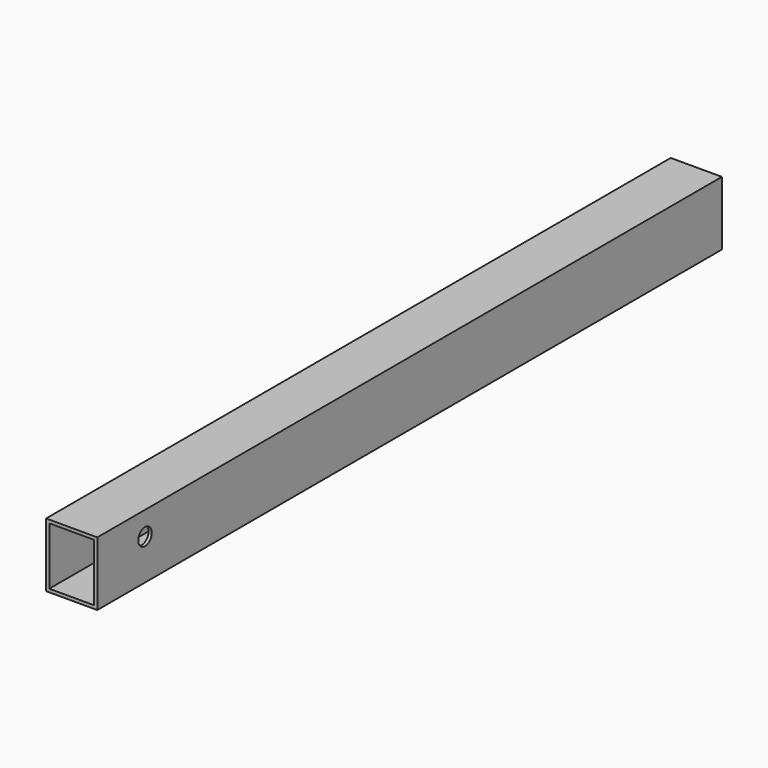
from build123d import *

# Parameters (mm, degrees)
F0_W          = 101.6
F0_H          = 127
F0_W_2        = 88.9
F0_H_2        = 114.3
F1_DEPTH      = 1524
F1_DEPTH_BACK = 25.4
F2_R          = 16.764
F3_DEPTH      = 127


# Not quite as in the source:
# - a feature names something its author has since deleted; it is built from what else it names


with BuildPart() as f1:
    # F0 (on Front) → F1 (new body, two sides)
    with BuildSketch(Plane.XZ) as f1_sk:
        with Locations((-14.2066246522, 5.0925366492)):
            Rectangle(F0_W, F0_H)
        with Locations((-14.2066246522, 5.0925366492)):
            Rectangle(F0_W_2, F0_H_2, mode=Mode.SUBTRACT)
    extrude(amount=F1_DEPTH)
    extrude(f1_sk.sketch, amount=-F1_DEPTH_BACK)

    # F2 (on face) → F3 (cut)
    with BuildSketch(Plane.YZ.offset(36.5933753478)):
        with Locations((-1405.636, 21.8565366492)):
            Circle(F2_R)
    extrude(amount=-F3_DEPTH, mode=Mode.SUBTRACT)


solid = f1.part
